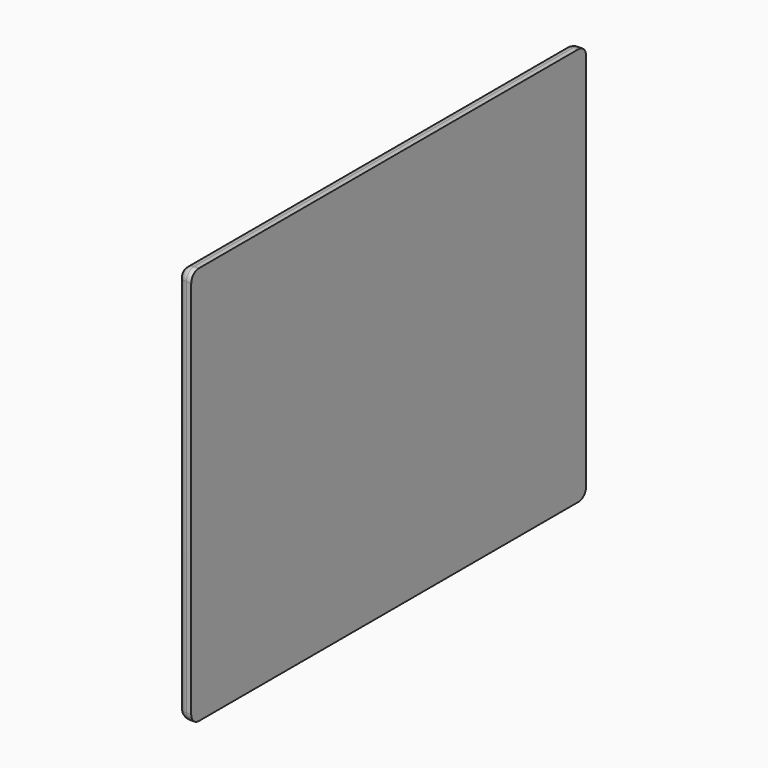
from build123d import *

# Parameters (mm, degrees)
F0_W     = 660.4
F0_H     = 533.4
F1_DEPTH = 19.05
F3_R     = 12.7


# Not quite as in the source:
# - two fillets or chamfers of one size are made in one step
# - a feature of the source that left no trace in its solid (it failed there, or was rolled back) is left out


with BuildPart() as f1:
    # F0 (on Right) → F1 (new body)
    with BuildSketch(Plane.YZ):
        with Locations((-50.8608140139, 1.481294632)):
            Rectangle(F0_W, F0_H)
    extrude(amount=F1_DEPTH)

    # F3
    f3_edges = [f1.edges().sort_by_distance(p)[0] for p in [
        (9.525, -381.060814, 268.181295),
        (9.525, -381.060814, -265.218705),
        (0, -381.060814, 1.481295),
        (9.525, 279.339186, -265.218705),
        (0, -50.860814, -265.218705),
        (9.525, 279.339186, 268.181295),
        (0, 279.339186, 1.481295),
        (0, -50.860814, 268.181295),
    ]]
    fillet(f3_edges, radius=F3_R)


solid = f1.part
